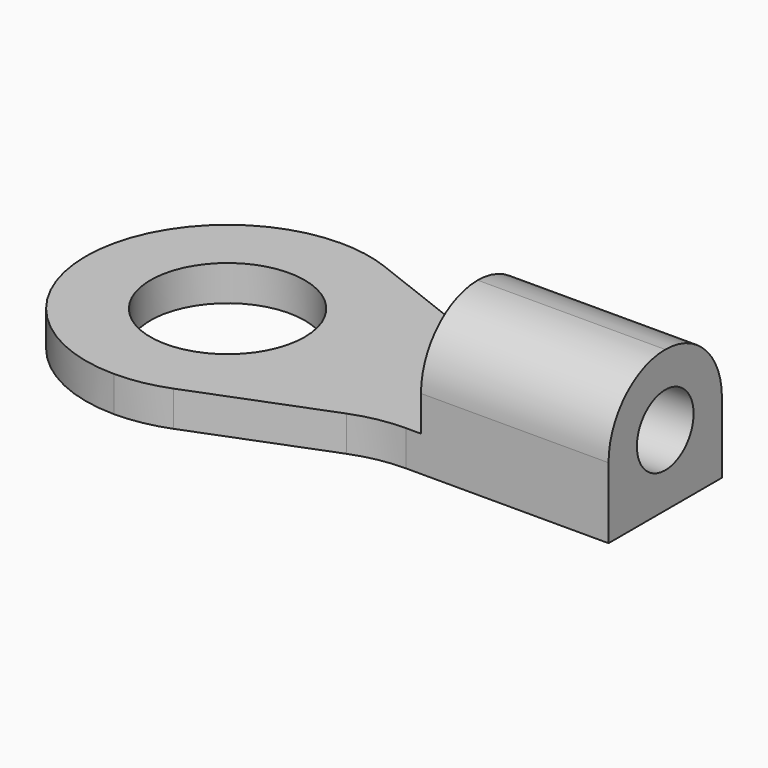
from build123d import *

# Parameters (mm, degrees)
F0_R     = 1.85
F1_DEPTH = 0.85
F2_W     = 4.5
F2_H     = 3.4
F3_DEPTH = 2.55
F4_R     = 1.69999
F5_R     = 0.85
F6_DEPTH = 25


# Not quite as in the source:
# - a fillet or chamfer is up to 0.001 mm smaller than in the source, because OpenCascade refuses the exact size


with BuildPart() as f1:
    # F0 (on Top) → F1 (new body)
    with BuildSketch(Plane.XY):
        with BuildLine():
            Line((9.0393070198, 1.7), (13.9, 1.7))
            Line((13.9, 1.7), (13.9, 5.1))
            Line((13.9, 5.1), (9.0393070198, 5.1))
            ThreePointArc((9.0393070198, 5.1), (8.4110104984, 5.1585566769), (7.8043557161, 5.332209717))
            Line((7.8043557161, 5.332209717), (4.6349513038, 6.567790283))
            ThreePointArc((4.6349513038, 6.567790283), (4.0282965214, 6.7414433231), (3.4, 6.8))
            ThreePointArc((3.4, 6.8), (0.995836944, 5.804163056), (0, 3.4))
            ThreePointArc((0, 3.4), (0.995836944, 0.995836944), (3.4, 0))
            ThreePointArc((3.4, 0), (4.0282965214, 0.0585566769), (4.6349513038, 0.232209717))
            Line((4.6349513038, 0.232209717), (7.8043557161, 1.467790283))
            ThreePointArc((7.8043557161, 1.467790283), (8.4110104984, 1.6414433231), (9.0393070198, 1.7))
        make_face()
        with Locations((3.4, 3.4)):
            Circle(F0_R, mode=Mode.SUBTRACT)
    extrude(amount=F1_DEPTH)

    # F2 (on face) → F3 (join)
    with BuildSketch(Plane.XY.offset(0.85)):
        with Locations((11.65, 3.4)):
            Rectangle(F2_W, F2_H)
    extrude(amount=F3_DEPTH)

    # F4 (radius 1.7 in the source; OpenCascade refuses exactly that, so slightly less here)
    f4_edges = [f1.edges().sort_by_distance(p)[0] for p in [
        (11.65, 5.1, 3.4),
        (11.65, 1.7, 3.4),
    ]]
    fillet(f4_edges, radius=F4_R)

    # F5 (on face) → F6 (cut)
    with BuildSketch(Plane.YZ.offset(13.9)):
        with Locations((3.4, 1.7)):
            Circle(F5_R)
    extrude(amount=-F6_DEPTH, mode=Mode.SUBTRACT)


solid = f1.part
